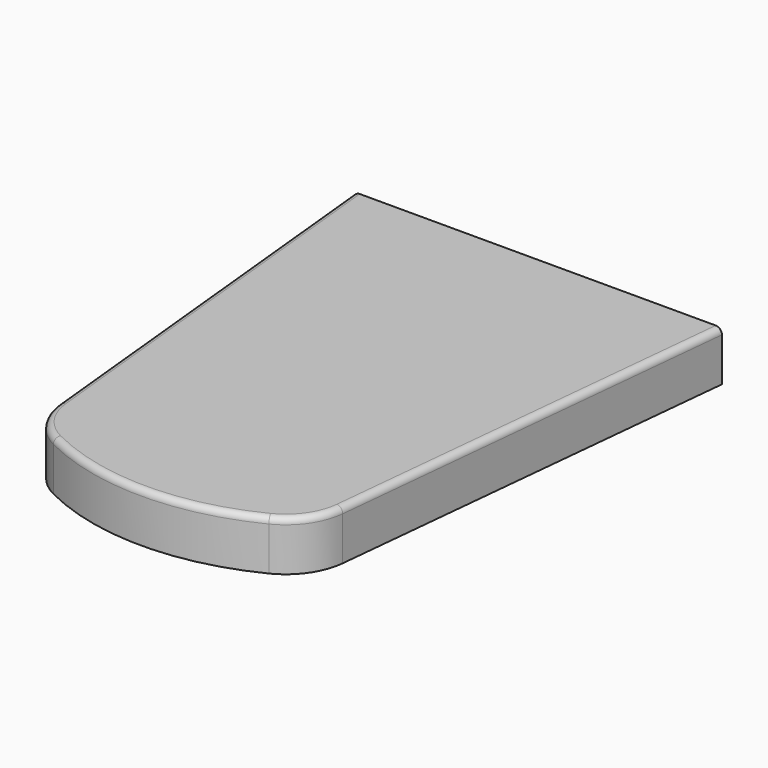
from build123d import *

# Parameters (mm, degrees)
F1_DEPTH = 5.08
F2_R     = 0.635


# Not quite as in the source:
# - a feature names something its author has since deleted; it is built from what else it names


with BuildPart() as f1:
    # F0 (on Top) → F1 (new body)
    with BuildSketch(Plane.XY):
        with BuildLine():
            Line((3.7253e-06, 50.8), (4.3267840925, 7.8043183677))
            ThreePointArc((4.3267840925, 7.8043183677), (5.4175944315, 4.8348440923), (7.8057635016, 2.7601650422))
            ThreePointArc((7.8057635016, 2.7601650422), (18.8061487686, 0.162150538), (29.8082212267, 2.753010822))
            ThreePointArc((29.8082212267, 2.753010822), (32.2000000346, 4.8294123123), (33.2912774596, 7.8028215671))
            Line((33.2912774596, 7.8028215671), (37.5920037253, 50.8))
            Line((37.5920037253, 50.8), (3.7253e-06, 50.8))
        make_face()
    extrude(amount=F1_DEPTH)

    # F2
    f2_edges = [f1.edges().sort_by_distance(p)[0] for p in [
        (18.806149, 0.162151, 5.08),
        (32.2, 4.829412, 5.08),
        (35.441641, 29.301411, 5.08),
        (2.163394, 29.302159, 5.08),
        (5.417594, 4.834844, 5.08),
    ]]
    fillet(f2_edges, radius=F2_R)


solid = f1.part
